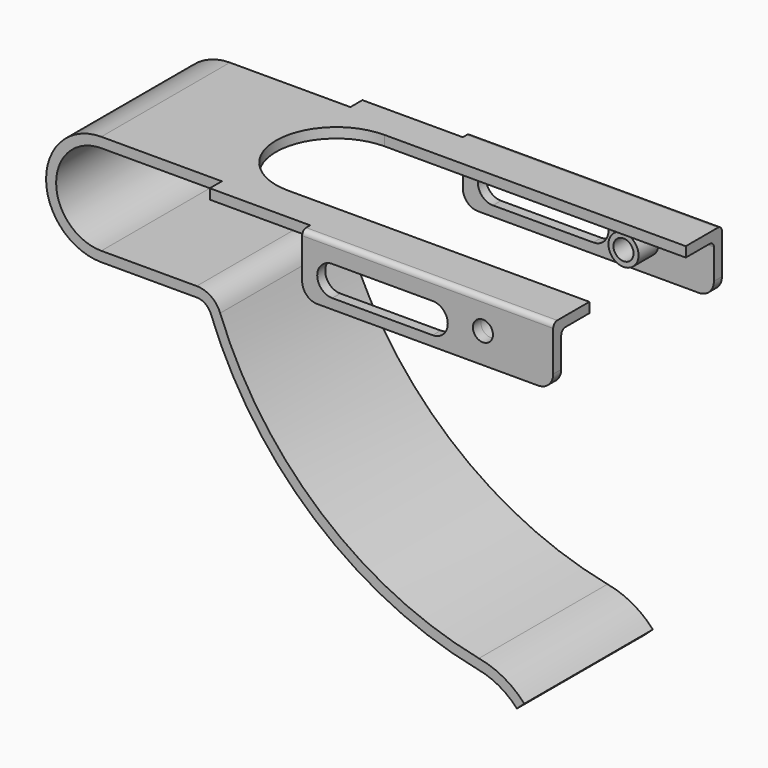
from build123d import *

# Parameters (mm, degrees)
F1_DEPTH  = 16
F2_W      = 70
F2_H      = 3
F3_DEPTH  = 2
F4_W      = 50
F4_H      = 12
F5_DEPTH  = 2
F6_R      = 1
F9_DEPTH  = 2
F11_DEPTH = 42.001
F13_D     = 4
F14_R     = 3
F14_R_2   = 2
F15_DEPTH = 5
F16_R     = 3


# Not quite as in the source:
# - a pattern or mirror of a feature is missing from the dataset's text; its kind, count and spacing are read off the source's solid


with BuildPart() as f1:
    # F0 (on Front) → F1 (new body)
    with BuildSketch(Plane.XZ):
        with BuildLine():
            ThreePointArc((0, -9), (-9, 0), (0, 9))
            Line((0, 9), (94, 9))
            Line((94, 9), (94, 11))
            Line((94, 11), (0, 11))
            ThreePointArc((0, 11), (-11, 0), (0, -11))
            Line((0, -11), (19, -11))
            ThreePointArc((19, -11), (20.704090422, -11.530976745), (21.8049592536, -12.9359494441))
            ThreePointArc((21.8049592536, -12.9359494441), (42.5173607247, -42.2788136793), (74.8275397389, -57.9651003113))
            ThreePointArc((74.8275397389, -57.9651003113), (79.1628330842, -59.4937576212), (82.7692987656, -62.344190369))
            Line((82.7692987656, -62.344190369), (84.2502282886, -61))
            ThreePointArc((84.2502282886, -61), (80.1403113626, -57.7488524545), (75.200382963, -56))
            ThreePointArc((75.200382963, -56), (43.8025480023, -40.74634786), (23.6749320894, -12.2265824069))
            ThreePointArc((23.6749320894, -12.2265824069), (21.8401507033, -9.8849612416), (19, -9))
            Line((19, -9), (0, -9))
        make_face()
    extrude(amount=F1_DEPTH)

    # F2 (on face) → F3 (join)
    with BuildSketch(Plane.XY.offset(11)):
        with Locations((59, -17.5)):
            Rectangle(F2_W, F2_H)
    extrude(amount=-F3_DEPTH)

    # F4 (on face) → F5 (join)
    with BuildSketch(Plane.XZ.offset(19)):
        with Locations((69, 5)):
            Rectangle(F4_W, F4_H)
    extrude(amount=F5_DEPTH)

    # F6
    f6_edges = [f1.edges().sort_by_distance(p)[0] for p in [
        (69, -21, 11),
        (69, -19, 9),
    ]]
    fillet(f6_edges, radius=F6_R)

    # F7: F1 across plane


with BuildPart() as f1_1:
    add(f1.part)
    add(f1.part.mirror(Plane.XZ))

    # F8 (on face) → F9 (cut)
    with BuildSketch(Plane.XY.offset(11)):
        with BuildLine():
            Line((94, 12), (34, 12))
            ThreePointArc((34, 12), (22, 0), (34, -12))
            Line((34, -12), (94, -12))
            Line((94, -12), (94, 12))
        make_face()
    extrude(amount=-F9_DEPTH, mode=Mode.SUBTRACT)

    # F10 (on face) → F11 (cut, through all)
    with BuildSketch(Plane.XZ.offset(21)):
        with BuildLine():
            ThreePointArc((50, 7), (47, 4), (50, 1))
            Line((50, 1), (70, 1))
            ThreePointArc((70, 1), (73, 4), (70, 7))
            Line((70, 7), (50, 7))
        make_face()
    extrude(amount=-F11_DEPTH, mode=Mode.SUBTRACT)

    # F13 (through all)
    with Locations(Plane.XZ.offset(21)):
        with Locations((80, 5)):
            Hole(F13_D / 2)

    # F14 (on face) → F15 (join)
    with BuildSketch(Plane(origin=(0, -19, 0), x_dir=(-1, 0, 0), z_dir=(0, 1, 0))):
        with Locations((-80, 5)):
            Circle(F14_R)
        with Locations((-80, 5)):
            Circle(F14_R_2, mode=Mode.SUBTRACT)
    f15 = extrude(amount=F15_DEPTH)

    # F15_copies: F15 across plane
    add(f15.mirror(Plane.ZX))

    # F16
    f16_edges = [f1_1.edges().sort_by_distance(p)[0] for p in [
        (94, -20, -1),
        (94, 20, -1),
        (44, 20, -1),
        (44, -20, -1),
    ]]
    fillet(f16_edges, radius=F16_R)


solid = f1_1.part
